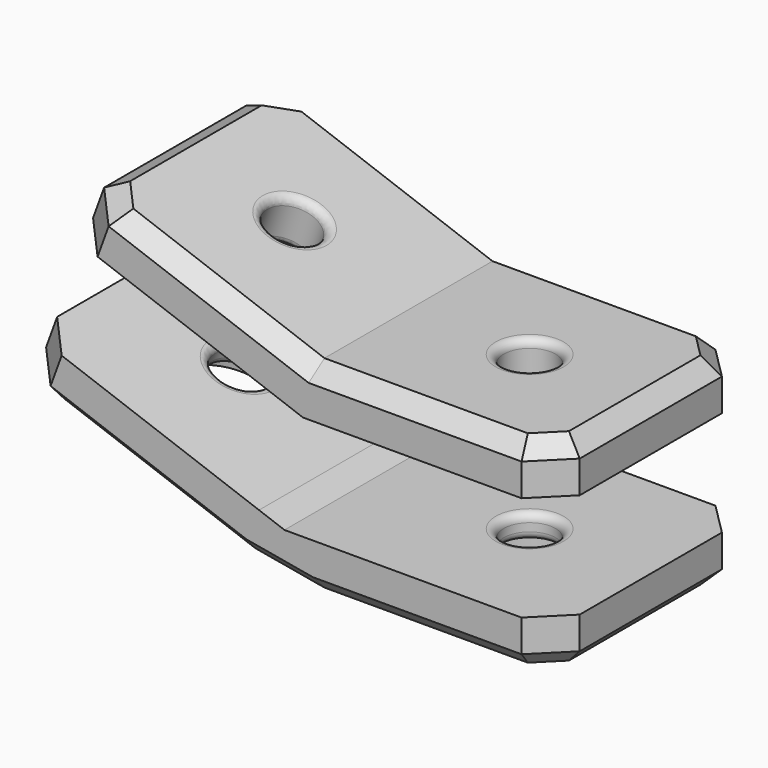
from build123d import *

# Parameters (mm, degrees)
F0_W           = 15
F0_H           = 3
F1_DEPTH       = 15
F2_R           = 1.6
F3_DEPTH       = 25
F4_R           = 1.6
F5_DEPTH       = 25
F7_DEPTH       = 25
F8_R           = 3.25
F8_R_2         = 1.6
F9_DEPTH       = 1.5
F10_R          = 3.25
F10_R_2        = 1.6
F11_DEPTH      = 1.5
F12_C1_SIZE    = 2
F12_C2_SIZE    = 2
F12_C3_SIZE    = 2
F12_C4_SIZE    = 2
F12_S1_C1_SIZE = 2
F12_S1_C2_SIZE = 2
F12_S1_C3_SIZE = 2
F12_S1_C4_SIZE = 2
F13_SIZE       = 1
F14_R          = 0.5
F15_SIZE       = 1


with BuildPart() as f1:
    # F0 (on Front) → F1 (new body)
    with BuildSketch(Plane.XZ):
        Polygon((-1.02606043, -2.8190778624), (0, 0), (-14.0953893118, 5.1303021499), (-15.1214497418, 2.3112242875), align=None)
        Polygon((0, -3), (0, 0), (-1.02606043, -2.8190778624), (-3.2491913616, -8.9270798975), (-4.2752517916, -11.7461577598), (0, -12.5), (0, -9.5), align=None)
        with Locations((7.5, -1.5)):
            Rectangle(F0_W, F0_H)
        Polygon((-4.2752517916, -11.7461577598), (-3.2491913616, -8.9270798975), (-17.3445806734, -3.7967777476), (-18.3706411034, -6.6158556099), align=None)
        with Locations((7.5, -11)):
            Rectangle(F0_W, F0_H)
    extrude(amount=F1_DEPTH)

    # F2 (on face) → F3 (cut)
    with BuildSketch(Plane(origin=(0, 0, 0), x_dir=(0.9396926208, 0, -0.3420201433), z_dir=(0.3420201433, 0, 0.9396926208))):
        with Locations((-7.5, -7.5)):
            Circle(F2_R)
    extrude(amount=-F3_DEPTH, mode=Mode.SUBTRACT)

    # F4 (on face) → F5 (cut)
    with BuildSketch(Plane.XY):
        with Locations((7.5, -7.5)):
            Circle(F4_R)
    extrude(amount=-F5_DEPTH, mode=Mode.SUBTRACT)

    # F6 (on face) → F7 (cut)
    with BuildSketch(Plane.XZ.offset(15)):
        Polygon((-1.6751063167, -9.5), (-0.5289809421, -3), (-1.02606043, -2.8190778624), (-3.2491913616, -8.9270798975), align=None)
        Polygon((0, -3), (-0.5289809421, -3), (-1.6751063167, -9.5), (0, -9.5), align=None)
    extrude(amount=-F7_DEPTH, mode=Mode.SUBTRACT)

    # F8 (on face) → F9 (cut)
    with BuildSketch(Plane(origin=(-4.2752517916, 0, -11.7461577598), x_dir=(0.9396926208, 0, -0.3420201433), z_dir=(-0.3420201433, 0, -0.9396926208))):
        with Locations((-7.5, 7.5)):
            Circle(F8_R)
        with Locations((-7.5, 7.5)):
            Circle(F8_R_2, mode=Mode.SUBTRACT)
    extrude(amount=-F9_DEPTH, mode=Mode.SUBTRACT)

    # F10 (on face) → F11 (cut)
    with BuildSketch(Plane(origin=(0, 0, -12.5), x_dir=(1, 0, 0), z_dir=(0, 0, -1))):
        with Locations((7.5, 7.5)):
            Circle(F10_R)
        with Locations((7.5, 7.5)):
            Circle(F10_R_2, mode=Mode.SUBTRACT)
    extrude(amount=-F11_DEPTH, mode=Mode.SUBTRACT)

    # F12: chamfer of 2 on 4 edges, made by hand

    # F12_c1
    f12_c1_edges = [f1.edges().sort_by_distance(p)[0] for p in [
        (15, 0, -1.5),
    ]]
    chamfer(f12_c1_edges, length=F12_C1_SIZE)

    # F12_c2
    f12_c2_edges = [f1.edges().sort_by_distance(p)[0] for p in [
        (15, -15, -1.5),
    ]]
    chamfer(f12_c2_edges, length=F12_C2_SIZE)

    # F12_c3
    f12_c3_edges = [f1.edges().sort_by_distance(p)[0] for p in [
        (-14.6084195268, 0, 3.7207632187),
    ]]
    chamfer(f12_c3_edges, length=F12_C3_SIZE)

    # F12_c4
    f12_c4_edges = [f1.edges().sort_by_distance(p)[0] for p in [
        (-14.6084195268, -15, 3.7207632187),
    ]]
    chamfer(f12_c4_edges, length=F12_C4_SIZE)

    # F12#s1: chamfer of 2 on 4 edges, made by hand

    # F12_s1_c1
    f12_s1_c1_edges = [f1.edges().sort_by_distance(p)[0] for p in [
        (-17.8576108884, 0, -5.2063166788),
    ]]
    chamfer(f12_s1_c1_edges, length=F12_S1_C1_SIZE)

    # F12_s1_c2
    f12_s1_c2_edges = [f1.edges().sort_by_distance(p)[0] for p in [
        (15, 0, -11),
    ]]
    chamfer(f12_s1_c2_edges, length=F12_S1_C2_SIZE)

    # F12_s1_c3
    f12_s1_c3_edges = [f1.edges().sort_by_distance(p)[0] for p in [
        (-17.8576108884, -15, -5.2063166788),
    ]]
    chamfer(f12_s1_c3_edges, length=F12_S1_C3_SIZE)

    # F12_s1_c4
    f12_s1_c4_edges = [f1.edges().sort_by_distance(p)[0] for p in [
        (15, -15, -11),
    ]]
    chamfer(f12_s1_c4_edges, length=F12_S1_C4_SIZE)

    # F13
    f13_edges = [f1.edges().sort_by_distance(p)[0] for p in [
        (-18.370641, -7.5, -6.615856),
        (-17.430948, -14, -6.957876),
        (-10.383254, -15, -9.523027),
        (-17.430948, -1, -6.957876),
        (-10.383254, 0, -9.523027),
        (-2.137626, 0, -12.123079),
        (-2.137626, -15, -12.123079),
        (6.5, -15, -12.5),
        (6.5, 0, -12.5),
        (14, -1, -12.5),
        (15, -7.5, -12.5),
        (14, -14, -12.5),
    ]]
    chamfer(f13_edges, length=F13_SIZE)

    # F14
    f14_edges = [f1.edges().sort_by_distance(p)[0] for p in [
        (-12.313424, -7.5, -7.224236),
        (5.9, -7.5, -11),
        (5.9, -7.5, -9.5),
        (-11.800394, -7.5, -5.814697),
        (-8.551203, -7.5, 3.112383),
        (5.9, -7.5, 0),
        (-9.577263, -7.5, 0.293305),
        (5.9, -7.5, -3),
    ]]
    fillet(f14_edges, radius=F14_R)

    # F15
    f15_edges = [f1.edges().sort_by_distance(p)[0] for p in [
        (-6.108002, -15, 2.223131),
        (6.5, -15, 0),
        (14, -14, 0),
        (15, -7.5, 0),
        (14, -1, 0),
        (6.5, 0, 0),
        (-6.108002, 0, 2.223131),
        (-13.155697, -14, 4.788282),
        (-14.095389, -7.5, 5.130302),
        (-13.155697, -1, 4.788282),
    ]]
    chamfer(f15_edges, length=F15_SIZE)


solid = f1.part
